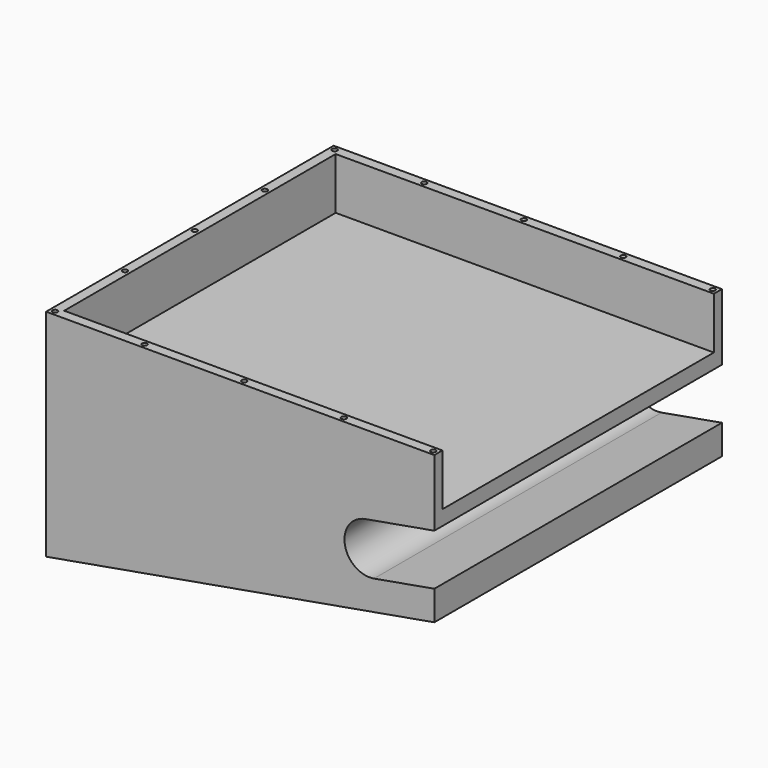
from build123d import *

# Parameters (mm, degrees)
F0_W      = 270
F0_H      = 250
F4_REACH  = 517.9673898595
F5_W      = 263
F5_H      = 236
F6_DEPTH  = 36
F8_DEPTH  = 250.001
F10_D     = 3.5
F10_DEPTH = 12
F10_TIP   = 1.0515060833


with BuildPart() as f4:
    f4_end = Plane(origin=(25.6515107494, 0, -145.4769465589), x_dir=(0.984807753, 0, 0.1736481777), z_dir=(-0.1736481777, 0, 0.984807753))
    # F0 (on Top) → F4 (new body, up to a plane its end follows)
    with BuildSketch(Plane.XY):
        with Locations((135, 125)):
            Rectangle(F0_W, F0_H)
    f4_long = extrude(amount=-F4_REACH, mode=Mode.PRIVATE)
    add(split(f4_long, bisect_by=f4_end, keep=Keep.TOP, mode=Mode.PRIVATE))

    # F5 (on face) → F6 (cut)
    with BuildSketch(Plane.XY):
        with Locations((138.5, 125)):
            Rectangle(F5_W, F5_H)
    extrude(amount=-F6_DEPTH, mode=Mode.SUBTRACT)

    # F7 (on face) → F8 (cut, through all)
    with BuildSketch(Plane.XZ):
        with BuildLine():
            Line((270, -46.2953201601), (221.9611568908, -54.7658643223))
            ThreePointArc((221.9611568908, -54.7658643223), (207.7658643223, -75.0388431092), (228.0388431092, -89.2341356777))
            Line((228.0388431092, -89.2341356777), (270, -81.8352515761))
            Line((270, -81.8352515761), (270, -46.2953201601))
        make_face()
    extrude(amount=-F8_DEPTH, mode=Mode.SUBTRACT)

    # F10
    with Locations(Plane.XY):
        with Locations((3.5, 64.25), (3.5, 125), (3.5, 185.75), (3.5, 246.5), (3.5, 3.5), (65.75, 3.5), (135, 3.5), (204.25, 3.5), (266.5, 3.5), (266.500000929, 246.5237677097), (204.25, 246.5237677097), (135, 246.5237677097), (65.75, 246.5)):
            Hole(F10_D / 2, depth=F10_DEPTH)
            with Locations((0, 0, -(F10_DEPTH + F10_TIP / 2))):  # 118° drill point
                Cone(0, F10_D / 2, F10_TIP, mode=Mode.SUBTRACT)


solid = f4.part
